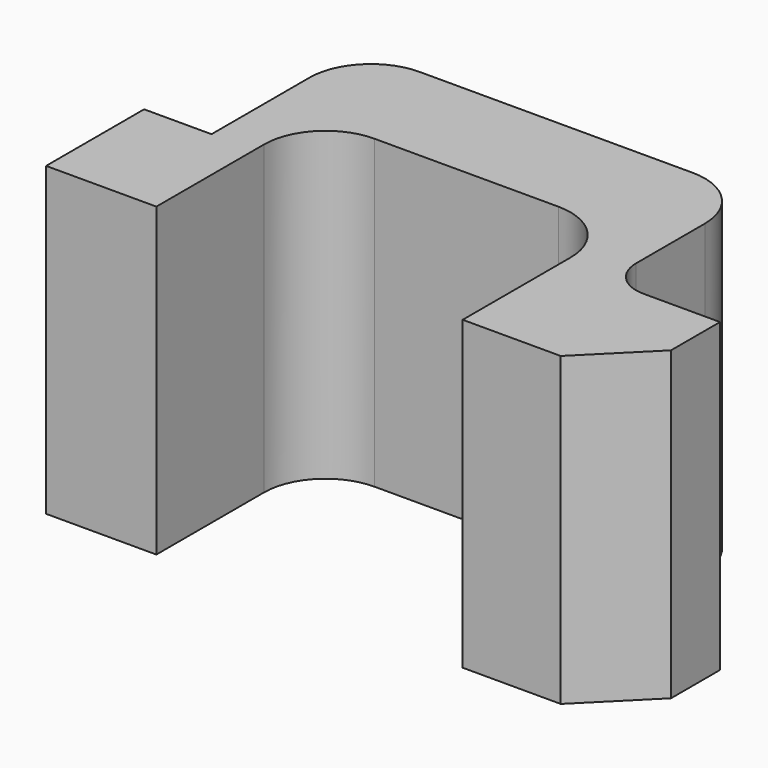
from build123d import *

# Parameters (mm, degrees)
F1_DEPTH = 25
F2_R     = 5
F3_R     = 3
F4_SIZE  = 5


with BuildPart() as f1:
    # F0 (on Top) → F1 (new body)
    with BuildSketch(Plane.XY):
        Polygon((0, 15), (-3.5, 15), (-3.5, 0), (-9, 0), (-9, -10), (0, -10), (0, 0), (0, 6), (25, 6), (25, 0), (25, -10), (38, -10), (38, 0), (28.7611037493, 0), (28.7611037493, 15), (25, 15), align=None)
    extrude(amount=F1_DEPTH)

    # F2
    f2_edges = [f1.edges().sort_by_distance(p)[0] for p in [
        (-3.5, 15, 12.5),
        (28.761104, 15, 12.5),
        (0, 6, 12.5),
        (25, 6, 12.5),
    ]]
    fillet(f2_edges, radius=F2_R)

    # F3
    f3_edges = [f1.edges().sort_by_distance(p)[0] for p in [
        (28.761104, 0, 12.5),
    ]]
    fillet(f3_edges, radius=F3_R)

    # F4
    f4_edges = [f1.edges().sort_by_distance(p)[0] for p in [
        (38, -10, 12.5),
    ]]
    chamfer(f4_edges, length=F4_SIZE)


solid = f1.part
